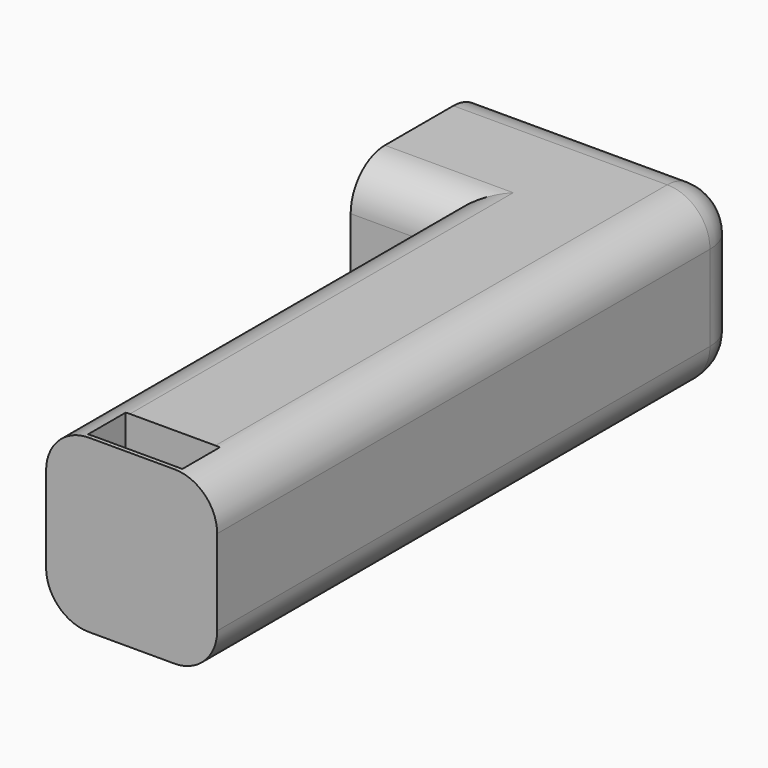
from build123d import *

# Parameters (mm, degrees)
F1_DEPTH     = 20
F2_DEPTH     = 5
F3_R         = 4.75
F4_DEPTH     = 10
F5_R         = 1.4
F6_DEPTH     = 5.4620024133
F7_T1_DEPTH  = 37.5
F7_T3_DEPTH  = 22.5
F7_T5_DEPTH  = 69.5
F7_T7_DEPTH  = 84.5
F7_T9_DEPTH  = 10
F7_S13_W     = 5
F7_S13_H     = 5
F7_T14_DEPTH = 5
F7_S19_W     = 5
F7_S19_H     = 5
F7_T20_DEPTH = 5
F7_T27_DEPTH = 35
F7_T31_DEPTH = 82
F7_T38_DEPTH = 35
F7_T42_DEPTH = 82


# Not quite as in the source:
# - a fillet or chamfer that OpenCascade refuses, or shapes differently, is made with other operations: its cross-section is extruded or revolved along the edge and cut away or added


with BuildPart() as f1:
    # F0 (on Top) → F1 (new body)
    with BuildSketch(Plane.XY):
        Polygon((0, 10), (0, 0), (0, -10), (10, -10), (10, -67), (30, -67), (30, 10), align=None)
        Polygon((25.5, -61), (25.5, -66.5), (20, -66.5), (14.5, -66.5), (14.5, -61), align=None, mode=Mode.SUBTRACT)
    extrude(amount=F1_DEPTH)

    # F0 (on Top) → F2 (join)
    with BuildSketch(Plane.XY):
        Polygon((20, -66.5), (25.5, -66.5), (25.5, -61), (14.5, -61), (14.5, -66.5), align=None)
    extrude(amount=F2_DEPTH)

    # F3 (on face) → F4 (cut)
    with BuildSketch(Plane(origin=(0, 0, 0), x_dir=(0, -1, 0), z_dir=(-1, 0, 0))):
        with Locations((0, 10)):
            Circle(F3_R)
    extrude(amount=-F4_DEPTH, mode=Mode.SUBTRACT)

    # F5 (on face) → F6 (cut, through all)
    with BuildSketch(Plane(origin=(0, 10, 0), x_dir=(-1, 0, 0), z_dir=(0, 1, 0))):
        with Locations((-5, 10)):
            Circle(F5_R)
    extrude(amount=-F6_DEPTH, mode=Mode.SUBTRACT)

    # F7: fillet of radius 5 on 9 edges, made by hand

    # F7_s2 → F7_t1 (cut)
    with BuildSketch(Plane.YZ.offset(-12.5)):
        with BuildLine():
            ThreePointArc((10, 15), (8.5355339059, 18.5355339059), (5, 20))
            Line((5, 20), (10, 20))
            Line((10, 20), (10, 15))
        make_face()
        with BuildLine():
            ThreePointArc((10, 5), (8.5355339059, 1.4644660941), (5, 0))
            Line((5, 0), (10, 0))
            Line((10, 0), (10, 5))
        make_face()
    extrude(amount=F7_T1_DEPTH, mode=Mode.SUBTRACT)

    # F7_s4 → F7_t3 (cut)
    with BuildSketch(Plane.YZ.offset(-12.5)):
        with BuildLine():
            ThreePointArc((-5, 20), (-8.5355339059, 18.5355339059), (-10, 15))
            Line((-10, 15), (-10, 20))
            Line((-10, 20), (-5, 20))
        make_face()
        with BuildLine():
            ThreePointArc((-5, 0), (-8.5355339059, 1.4644660941), (-10, 5))
            Line((-10, 5), (-10, 0))
            Line((-10, 0), (-5, 0))
        make_face()
    extrude(amount=F7_T3_DEPTH, mode=Mode.SUBTRACT)

    # F7_s6 → F7_t5 (cut)
    with BuildSketch(Plane.XZ.offset(10)):
        with BuildLine():
            ThreePointArc((15, 20), (11.4644660941, 18.5355339059), (10, 15))
            Line((10, 15), (10, 20))
            Line((10, 20), (15, 20))
        make_face()
        with BuildLine():
            ThreePointArc((15, 0), (11.4644660941, 1.4644660941), (10, 5))
            Line((10, 5), (10, 0))
            Line((10, 0), (15, 0))
        make_face()
    extrude(amount=F7_T5_DEPTH, mode=Mode.SUBTRACT)

    # F7_s8 → F7_t7 (cut)
    with BuildSketch(Plane.XZ.offset(-5)):
        with BuildLine():
            ThreePointArc((25, 20), (28.5355339059, 18.5355339059), (30, 15))
            Line((30, 15), (30, 20))
            Line((30, 20), (25, 20))
        make_face()
        with BuildLine():
            ThreePointArc((25, 0), (28.5355339059, 1.4644660941), (30, 5))
            Line((30, 5), (30, 0))
            Line((30, 0), (25, 0))
        make_face()
    extrude(amount=F7_T7_DEPTH, mode=Mode.SUBTRACT)

    # F7_s10 → F7_t9 (cut)
    with BuildSketch(Plane.XY.offset(5)):
        with BuildLine():
            ThreePointArc((25, 10), (28.5355339059, 8.5355339059), (30, 5))
            Line((30, 5), (30, 10))
            Line((30, 10), (25, 10))
        make_face()
    extrude(amount=F7_T9_DEPTH, mode=Mode.SUBTRACT)


with BuildPart() as f7_tool12:
    # F7_s13 → F7_t14 (new body)
    with BuildSketch(Plane.XZ.offset(-5)):
        with Locations((27.5, 17.5)):
            Rectangle(F7_S13_W, F7_S13_H)
    extrude(amount=-F7_T14_DEPTH)

    # F7_s15 → F7_t16 (revolve, cut)
    with BuildSketch(Plane(origin=(25, 5, 15), x_dir=(-0.7071067812, 0, -0.7071067812), z_dir=(0.7071067812, 0, -0.7071067812))):
        with BuildLine():
            ThreePointArc((0, -5), (5, 0), (0, 5))
            Line((0, 5), (0, -5))
        make_face()
    revolve(axis=Axis((25, 5, 15), (0, 1, 0)), mode=Mode.SUBTRACT)


with BuildPart() as f1_1:
    add(f1.part)

    # F7_t11: cut F7_tool12
    add(f7_tool12.part, mode=Mode.SUBTRACT)


with BuildPart() as f7_tool18:
    # F7_s19 → F7_t20 (new body)
    with BuildSketch(Plane.XZ.offset(-5)):
        with Locations((27.5, 2.5)):
            Rectangle(F7_S19_W, F7_S19_H)
    extrude(amount=-F7_T20_DEPTH)

    # F7_s21 → F7_t22 (revolve, cut)
    with BuildSketch(Plane(origin=(25, 5, 5), x_dir=(-0.7071067812, 0, 0.7071067812), z_dir=(-0.7071067812, 0, -0.7071067812))):
        with BuildLine():
            ThreePointArc((0, -5), (5, 0), (0, 5))
            Line((0, 5), (0, -5))
        make_face()
    revolve(axis=Axis((25, 5, 5), (0, 1, 0)), mode=Mode.SUBTRACT)


with BuildPart() as f1_2:
    add(f1_1.part)

    # F7_t17: cut F7_tool18
    add(f7_tool18.part, mode=Mode.SUBTRACT)


with BuildPart() as f7_tool25:
    # F7_s26 → F7_t27 (new body)
    with BuildSketch(Plane.YZ.offset(-12.5)):
        with BuildLine():
            ThreePointArc((-5, 20), (-8.5355339059, 18.5355339059), (-10, 15))
            Line((-10, 15), (-10, 20))
            Line((-10, 20), (-5, 20))
        make_face()
    extrude(amount=F7_T27_DEPTH)

    split(bisect_by=Plane.YZ.offset(10), keep=Keep.TOP)


with BuildPart() as f7_tool29:
    # F7_s30 → F7_t31 (new body)
    with BuildSketch(Plane.XZ.offset(-2.5)):
        with BuildLine():
            ThreePointArc((15, 20), (11.4644660941, 18.5355339059), (10, 15))
            Line((10, 15), (10, 20))
            Line((10, 20), (15, 20))
        make_face()
    extrude(amount=F7_T31_DEPTH)

    split(bisect_by=Plane.XZ.offset(10), keep=Keep.BOTTOM)


with BuildPart() as f7_tool25_1:
    add(f7_tool25.part)

    # F7_t33: intersect F7_tool29
    add(f7_tool29.part, mode=Mode.INTERSECT)


with BuildPart() as f1_3:
    add(f1_2.part)

    # F7_t23: cut F7_tool25
    add(f7_tool25_1.part, mode=Mode.SUBTRACT)


with BuildPart() as f7_tool36:
    # F7_s37 → F7_t38 (new body)
    with BuildSketch(Plane.YZ.offset(-12.5)):
        with BuildLine():
            ThreePointArc((-5, 0), (-8.5355339059, 1.4644660941), (-10, 5))
            Line((-10, 5), (-10, 0))
            Line((-10, 0), (-5, 0))
        make_face()
    extrude(amount=F7_T38_DEPTH)

    split(bisect_by=Plane.YZ.offset(10), keep=Keep.TOP)


with BuildPart() as f7_tool40:
    # F7_s41 → F7_t42 (new body)
    with BuildSketch(Plane.XZ.offset(-2.5)):
        with BuildLine():
            ThreePointArc((15, 0), (11.4644660941, 1.4644660941), (10, 5))
            Line((10, 5), (10, 0))
            Line((10, 0), (15, 0))
        make_face()
    extrude(amount=F7_T42_DEPTH)

    split(bisect_by=Plane.XZ.offset(10), keep=Keep.BOTTOM)


with BuildPart() as f7_tool36_1:
    add(f7_tool36.part)

    # F7_t44: intersect F7_tool40
    add(f7_tool40.part, mode=Mode.INTERSECT)


with BuildPart() as f1_4:
    add(f1_3.part)

    # F7_t34: cut F7_tool36
    add(f7_tool36_1.part, mode=Mode.SUBTRACT)


solid = f1_4.part
